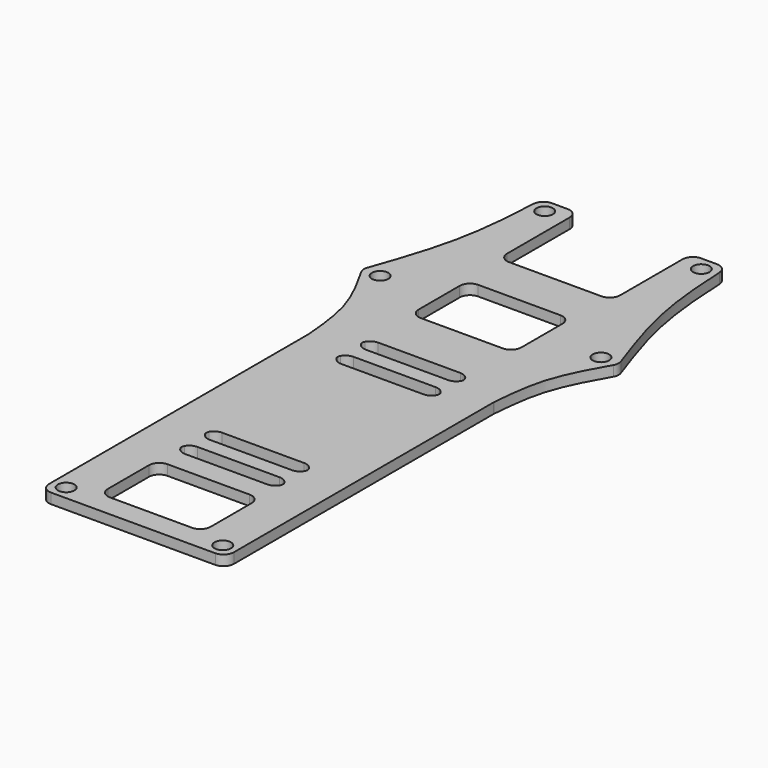
from build123d import *

# Parameters (mm, degrees)
F0_R          = 1.6
F0_W          = 20
F0_H          = 3
F0_H_2        = 14
F0_W_2        = 36
F0_H_3        = 50
F1_DEPTH      = 2
F2_T3_DEPTH   = 12
F2_T6_DEPTH   = 12
F2_T9_DEPTH   = 11.4916492708
F2_T12_DEPTH  = 11.4916492708
F2_T15_DEPTH  = 12
F2_T18_DEPTH  = 12
F2_T21_DEPTH  = 6.5584053931
F2_T24_DEPTH  = 6.5584053931
F2_T28_DEPTH  = 2
F2_T31_DEPTH  = 2
F2_T34_DEPTH  = 2
F2_T37_DEPTH  = 2
F2_T40_DEPTH  = 2
F2_T43_DEPTH  = 2
F2_T46_DEPTH  = 2
F2_T49_DEPTH  = 2
F2_T52_DEPTH  = 2
F2_T55_DEPTH  = 2
F2_T58_DEPTH  = 2
F2_T61_DEPTH  = 2
F2_T64_DEPTH  = 2
F2_T67_DEPTH  = 2
F2_T70_DEPTH  = 2
F2_T73_DEPTH  = 2
F2_T76_DEPTH  = 2
F2_T79_DEPTH  = 2
F2_T82_DEPTH  = 2
F2_T85_DEPTH  = 2
F2_T88_DEPTH  = 2
F2_T91_DEPTH  = 2
F2_T94_DEPTH  = 2
F2_T97_DEPTH  = 2
F2_T100_DEPTH = 2
F2_T103_DEPTH = 2
F2_T106_DEPTH = 2
F2_T109_DEPTH = 2
F3_R          = 1


# Not quite as in the source:
# - a fillet or chamfer that OpenCascade refuses, or shapes differently, is made with other operations: its cross-section is extruded or revolved along the edge and cut away or added
# - a feature names something its author has since deleted; it is built from what else it names


with BuildPart() as f1:
    # F0 (on Top) → F1 (new body)
    with BuildSketch(Plane.XY):
        Polygon((-11, 72), (-18, 72), (-18, 15.25), (-18, 0), (18, 0), (18, 15.25), (18, 72), (11, 72), (11, 52.774557963), (-11, 52.774557963), align=None)
        with Locations((-15.25, 69.25)):
            Circle(F0_R, mode=Mode.SUBTRACT)
        with Locations((0, 12.15)):
            Rectangle(F0_W, F0_H, mode=Mode.SUBTRACT)
        with Locations((0, 18.15)):
            Rectangle(F0_W, F0_H, mode=Mode.SUBTRACT)
        with Locations((0, 37)):
            Rectangle(F0_W, F0_H_2, mode=Mode.SUBTRACT)
        with Locations((15.25, 69.25)):
            Circle(F0_R, mode=Mode.SUBTRACT)
        with BuildLine():
            Line((-18, 15.25), (-18, 72))
            add(Edge.make_bspline(
                [(-18, 72), (-18.3026254462, 66.1394008634), (-18.9136987258, 54.305447113), (-22.9583868009, 42.805008272), (-25, 37)],
                knots=[0, 0, 0, 0, 0.4952359338, 1, 1, 1, 1], degree=3))
            add(Edge.make_bspline(
                [(-25, 37), (-22.9586488257, 33.418624871), (-18.967687527, 26.4168263973), (-18.3175811324, 18.9147918612), (-18, 15.25)],
                knots=[0, 0, 0, 0, 0.511493603, 1, 1, 1, 1], degree=3))
        make_face()
        with Locations((-21.5, 37)):
            Circle(F0_R, mode=Mode.SUBTRACT)
        with Locations((0, -25)):
            Rectangle(F0_W_2, F0_H_3)
        with Locations((-15.25, -47.25)):
            Circle(F0_R, mode=Mode.SUBTRACT)
        Polygon((10, -45.65), (0, -45.65), (-10, -45.65), (-10, -31.65), (0, -31.65), (10, -31.65), align=None, mode=Mode.SUBTRACT)
        with Locations((0, -25.85)):
            Rectangle(F0_W, F0_H, mode=Mode.SUBTRACT)
        with Locations((0, -19.85)):
            Rectangle(F0_W, F0_H, mode=Mode.SUBTRACT)
        with Locations((15.25, -47.25)):
            Circle(F0_R, mode=Mode.SUBTRACT)
        with BuildLine():
            Line((18, 72), (18, 15.25))
            add(Edge.make_bspline(
                [(25, 37), (22.9586488257, 33.418624871), (18.967687527, 26.4168263973), (18.3175811324, 18.9147918612), (18, 15.25)],
                knots=[0, 0, 0, 0, 0.511493603, 1, 1, 1, 1], degree=3))
            add(Edge.make_bspline(
                [(18, 72), (18.3026254462, 66.1394008634), (18.9136987258, 54.305447113), (22.9583868009, 42.805008272), (25, 37)],
                knots=[0, 0, 0, 0, 0.4952359338, 1, 1, 1, 1], degree=3))
        make_face()
        with Locations((21.5, 37)):
            Circle(F0_R, mode=Mode.SUBTRACT)
    extrude(amount=F1_DEPTH)

    # F2: fillet of radius 2 on 36 edges, made by hand


with BuildPart() as f2_tool1:
    # F2_s2 → F2_t3 (new body)
    with BuildSketch(Plane.XY.offset(-5)):
        with BuildLine():
            ThreePointArc((13, 72), (11.5857864376, 71.4142135624), (11, 70))
            Line((11, 70), (11, 72))
            Line((11, 72), (13, 72))
        make_face()
    extrude(amount=F2_T3_DEPTH)


with BuildPart() as f2_tool4:
    # F2_s5 → F2_t6 (new body)
    with BuildSketch(Plane.XY.offset(-5)):
        with BuildLine():
            ThreePointArc((-13, 72), (-11.5857864376, 71.4142135624), (-11, 70))
            Line((-11, 70), (-11, 72))
            Line((-11, 72), (-13, 72))
        make_face()
    extrude(amount=F2_T6_DEPTH)


with BuildPart() as f2_tool7:
    # F2_s8 → F2_t9 (new body)
    with BuildSketch(Plane.XY.offset(-4.7458246354)):
        with BuildLine():
            ThreePointArc((-16.1016701458, 72), (-17.4777245293, 71.4513698129), (-18.0988339389, 70.1064743339))
            ThreePointArc((-18.0988339389, 70.1064743339), (-18.0490214969, 71.0532165802), (-18, 72))
            Line((-18, 72), (-16.1016701458, 72))
        make_face()
    extrude(amount=F2_T9_DEPTH)


with BuildPart() as f2_tool10:
    # F2_s11 → F2_t12 (new body)
    with BuildSketch(Plane.XY.offset(-4.7458246354)):
        with BuildLine():
            ThreePointArc((18.0988339389, 70.1064743339), (17.4777245293, 71.4513698129), (16.1016701458, 72))
            Line((16.1016701458, 72), (18, 72))
            ThreePointArc((18, 72), (18.0490214969, 71.0532165802), (18.0988339389, 70.1064743339))
        make_face()
    extrude(amount=F2_T12_DEPTH)


with BuildPart() as f2_tool13:
    # F2_s14 → F2_t15 (new body)
    with BuildSketch(Plane.XY.offset(-5)):
        with BuildLine():
            ThreePointArc((-18, -48), (-17.4142135624, -49.4142135624), (-16, -50))
            Line((-16, -50), (-18, -50))
            Line((-18, -50), (-18, -48))
        make_face()
    extrude(amount=F2_T15_DEPTH)


with BuildPart() as f2_tool16:
    # F2_s17 → F2_t18 (new body)
    with BuildSketch(Plane.XY.offset(-5)):
        with BuildLine():
            ThreePointArc((16, -50), (17.4142135624, -49.4142135624), (18, -48))
            Line((18, -48), (18, -50))
            Line((18, -50), (16, -50))
        make_face()
    extrude(amount=F2_T18_DEPTH)


with BuildPart() as f2_tool19:
    # F2_s20 → F2_t21 (new body)
    with BuildSketch(Plane.XY.offset(-2.2792026965)):
        with BuildLine():
            ThreePointArc((-24.697621668, 37.8600754231), (-24.8026656547, 37.0182702368), (-24.5493168148, 36.2086502171))
            ThreePointArc((-24.5493168148, 36.2086502171), (-24.774551113, 36.6043862268), (-25, 37))
            ThreePointArc((-25, 37), (-24.8487744639, 37.4300249237), (-24.697621668, 37.8600754231))
        make_face()
    extrude(amount=F2_T21_DEPTH)


with BuildPart() as f2_tool22:
    # F2_s23 → F2_t24 (new body)
    with BuildSketch(Plane.XY.offset(-2.2792026965)):
        with BuildLine():
            ThreePointArc((24.5493168148, 36.2086502171), (24.8026656547, 37.0182702368), (24.697621668, 37.8600754231))
            ThreePointArc((24.697621668, 37.8600754231), (24.8487744639, 37.4300249237), (25, 37))
            ThreePointArc((25, 37), (24.774551113, 36.6043862268), (24.5493168148, 36.2086502171))
        make_face()
    extrude(amount=F2_T24_DEPTH)


with BuildPart() as f1_1:
    add(f1.part)

    # F2_t25: cut F2_tool1, F2_tool4, F2_tool7, F2_tool10, F2_tool13, F2_tool16, F2_tool19, F2_tool22
    add([f2_tool1.part, f2_tool4.part, f2_tool7.part, f2_tool10.part, f2_tool13.part, f2_tool16.part, f2_tool19.part, f2_tool22.part], mode=Mode.SUBTRACT)


with BuildPart() as f2_tool26:
    # F2_s27 → F2_t28 (new body)
    with BuildSketch(Plane.XY):
        with BuildLine():
            ThreePointArc((-11, 54.774557963), (-10.4142135624, 53.3603444006), (-9, 52.774557963))
            Line((-9, 52.774557963), (-11, 52.774557963))
            Line((-11, 52.774557963), (-11, 54.774557963))
        make_face()
    extrude(amount=F2_T28_DEPTH)


with BuildPart() as f2_tool29:
    # F2_s30 → F2_t31 (new body)
    with BuildSketch(Plane.XY):
        with BuildLine():
            ThreePointArc((9, 52.774557963), (10.4142135624, 53.3603444006), (11, 54.774557963))
            Line((11, 54.774557963), (11, 52.774557963))
            Line((11, 52.774557963), (9, 52.774557963))
        make_face()
    extrude(amount=F2_T31_DEPTH)


with BuildPart() as f2_tool32:
    # F2_s33 → F2_t34 (new body)
    with BuildSketch(Plane.XY):
        with BuildLine():
            ThreePointArc((18.0074697855, 15.3361946129), (18.001868319, 15.2499281672), (18, 15.1635002466))
            Line((18, 15.1635002466), (18, 15.25))
            ThreePointArc((18, 15.25), (18.0037347479, 15.293097319), (18.0074697855, 15.3361946129))
        make_face()
    extrude(amount=F2_T34_DEPTH)


with BuildPart() as f2_tool35:
    # F2_s36 → F2_t37 (new body)
    with BuildSketch(Plane.XY):
        with BuildLine():
            ThreePointArc((-18, 15.1635002466), (-18.001868319, 15.2499281672), (-18.0074697855, 15.3361946129))
            ThreePointArc((-18.0074697855, 15.3361946129), (-18.0037347479, 15.293097319), (-18, 15.25))
            Line((-18, 15.25), (-18, 15.1635002466))
        make_face()
    extrude(amount=F2_T37_DEPTH)


with BuildPart() as f2_tool38:
    # F2_s39 → F2_t40 (new body)
    with BuildSketch(Plane.XY):
        with BuildLine():
            ThreePointArc((10, 11.65), (9.4142135624, 13.0642135624), (8, 13.65))
            Line((8, 13.65), (10, 13.65))
            Line((10, 13.65), (10, 11.65))
        make_face()
    extrude(amount=F2_T40_DEPTH)


with BuildPart() as f2_tool41:
    # F2_s42 → F2_t43 (new body)
    with BuildSketch(Plane.XY):
        with BuildLine():
            ThreePointArc((-8, 13.65), (-9.4142135624, 13.0642135624), (-10, 11.65))
            Line((-10, 11.65), (-10, 13.65))
            Line((-10, 13.65), (-8, 13.65))
        make_face()
    extrude(amount=F2_T43_DEPTH)


with BuildPart() as f2_tool44:
    # F2_s45 → F2_t46 (new body)
    with BuildSketch(Plane.XY):
        with BuildLine():
            ThreePointArc((-8, 10.65), (-9.4142135624, 11.2357864376), (-10, 12.65))
            Line((-10, 12.65), (-10, 10.65))
            Line((-10, 10.65), (-8, 10.65))
        make_face()
    extrude(amount=F2_T46_DEPTH)


with BuildPart() as f2_tool47:
    # F2_s48 → F2_t49 (new body)
    with BuildSketch(Plane.XY):
        with BuildLine():
            ThreePointArc((10, 12.65), (9.4142135624, 11.2357864376), (8, 10.65))
            Line((8, 10.65), (10, 10.65))
            Line((10, 10.65), (10, 12.65))
        make_face()
    extrude(amount=F2_T49_DEPTH)


with BuildPart() as f2_tool50:
    # F2_s51 → F2_t52 (new body)
    with BuildSketch(Plane.XY):
        with BuildLine():
            ThreePointArc((8, -24.35), (9.4142135624, -24.9357864376), (10, -26.35))
            Line((10, -26.35), (10, -24.35))
            Line((10, -24.35), (8, -24.35))
        make_face()
    extrude(amount=F2_T52_DEPTH)


with BuildPart() as f2_tool53:
    # F2_s54 → F2_t55 (new body)
    with BuildSketch(Plane.XY):
        with BuildLine():
            ThreePointArc((-8, -24.35), (-9.4142135624, -24.9357864376), (-10, -26.35))
            Line((-10, -26.35), (-10, -24.35))
            Line((-10, -24.35), (-8, -24.35))
        make_face()
    extrude(amount=F2_T55_DEPTH)


with BuildPart() as f2_tool56:
    # F2_s57 → F2_t58 (new body)
    with BuildSketch(Plane.XY):
        with BuildLine():
            ThreePointArc((-10, -25.35), (-9.4142135624, -26.7642135624), (-8, -27.35))
            Line((-8, -27.35), (-10, -27.35))
            Line((-10, -27.35), (-10, -25.35))
        make_face()
    extrude(amount=F2_T58_DEPTH)


with BuildPart() as f2_tool59:
    # F2_s60 → F2_t61 (new body)
    with BuildSketch(Plane.XY):
        with BuildLine():
            ThreePointArc((10, -25.35), (9.4142135624, -26.7642135624), (8, -27.35))
            Line((8, -27.35), (10, -27.35))
            Line((10, -27.35), (10, -25.35))
        make_face()
    extrude(amount=F2_T61_DEPTH)


with BuildPart() as f2_tool62:
    # F2_s63 → F2_t64 (new body)
    with BuildSketch(Plane.XY):
        with BuildLine():
            ThreePointArc((-10, -33.65), (-9.4142135624, -32.2357864376), (-8, -31.65))
            Line((-8, -31.65), (-10, -31.65))
            Line((-10, -31.65), (-10, -33.65))
        make_face()
    extrude(amount=F2_T64_DEPTH)


with BuildPart() as f2_tool65:
    # F2_s66 → F2_t67 (new body)
    with BuildSketch(Plane.XY):
        with BuildLine():
            ThreePointArc((10, -33.65), (9.4142135624, -32.2357864376), (8, -31.65))
            Line((8, -31.65), (10, -31.65))
            Line((10, -31.65), (10, -33.65))
        make_face()
    extrude(amount=F2_T67_DEPTH)


with BuildPart() as f2_tool68:
    # F2_s69 → F2_t70 (new body)
    with BuildSketch(Plane.XY):
        with BuildLine():
            ThreePointArc((8, -45.65), (9.4142135624, -45.0642135624), (10, -43.65))
            Line((10, -43.65), (10, -45.65))
            Line((10, -45.65), (8, -45.65))
        make_face()
    extrude(amount=F2_T70_DEPTH)


with BuildPart() as f2_tool71:
    # F2_s72 → F2_t73 (new body)
    with BuildSketch(Plane.XY):
        with BuildLine():
            ThreePointArc((-8, -45.65), (-9.4142135624, -45.0642135624), (-10, -43.65))
            Line((-10, -43.65), (-10, -45.65))
            Line((-10, -45.65), (-8, -45.65))
        make_face()
    extrude(amount=F2_T73_DEPTH)


with BuildPart() as f2_tool74:
    # F2_s75 → F2_t76 (new body)
    with BuildSketch(Plane.XY):
        with BuildLine():
            ThreePointArc((-8, 19.65), (-9.4142135624, 19.0642135624), (-10, 17.65))
            Line((-10, 17.65), (-10, 19.65))
            Line((-10, 19.65), (-8, 19.65))
        make_face()
    extrude(amount=F2_T76_DEPTH)


with BuildPart() as f2_tool77:
    # F2_s78 → F2_t79 (new body)
    with BuildSketch(Plane.XY):
        with BuildLine():
            ThreePointArc((-10, 18.65), (-9.4142135624, 17.2357864376), (-8, 16.65))
            Line((-8, 16.65), (-10, 16.65))
            Line((-10, 16.65), (-10, 18.65))
        make_face()
    extrude(amount=F2_T79_DEPTH)


with BuildPart() as f2_tool80:
    # F2_s81 → F2_t82 (new body)
    with BuildSketch(Plane.XY):
        with BuildLine():
            ThreePointArc((-8, -21.35), (-9.4142135624, -20.7642135624), (-10, -19.35))
            Line((-10, -19.35), (-10, -21.35))
            Line((-10, -21.35), (-8, -21.35))
        make_face()
    extrude(amount=F2_T82_DEPTH)


with BuildPart() as f2_tool83:
    # F2_s84 → F2_t85 (new body)
    with BuildSketch(Plane.XY):
        with BuildLine():
            ThreePointArc((-8, -18.35), (-9.4142135624, -18.9357864376), (-10, -20.35))
            Line((-10, -20.35), (-10, -18.35))
            Line((-10, -18.35), (-8, -18.35))
        make_face()
    extrude(amount=F2_T85_DEPTH)


with BuildPart() as f2_tool86:
    # F2_s87 → F2_t88 (new body)
    with BuildSketch(Plane.XY):
        with BuildLine():
            ThreePointArc((10, -20.35), (9.4142135624, -18.9357864376), (8, -18.35))
            Line((8, -18.35), (10, -18.35))
            Line((10, -18.35), (10, -20.35))
        make_face()
    extrude(amount=F2_T88_DEPTH)


with BuildPart() as f2_tool89:
    # F2_s90 → F2_t91 (new body)
    with BuildSketch(Plane.XY):
        with BuildLine():
            ThreePointArc((10, -19.35), (9.4142135624, -20.7642135624), (8, -21.35))
            Line((8, -21.35), (10, -21.35))
            Line((10, -21.35), (10, -19.35))
        make_face()
    extrude(amount=F2_T91_DEPTH)


with BuildPart() as f2_tool92:
    # F2_s93 → F2_t94 (new body)
    with BuildSketch(Plane.XY):
        with BuildLine():
            ThreePointArc((10, 18.65), (9.4142135624, 17.2357864376), (8, 16.65))
            Line((8, 16.65), (10, 16.65))
            Line((10, 16.65), (10, 18.65))
        make_face()
    extrude(amount=F2_T94_DEPTH)


with BuildPart() as f2_tool95:
    # F2_s96 → F2_t97 (new body)
    with BuildSketch(Plane.XY):
        with BuildLine():
            ThreePointArc((8, 19.65), (9.4142135624, 19.0642135624), (10, 17.65))
            Line((10, 17.65), (10, 19.65))
            Line((10, 19.65), (8, 19.65))
        make_face()
    extrude(amount=F2_T97_DEPTH)


with BuildPart() as f2_tool98:
    # F2_s99 → F2_t100 (new body)
    with BuildSketch(Plane.XY):
        with BuildLine():
            ThreePointArc((-8, 44), (-9.4142135624, 43.4142135624), (-10, 42))
            Line((-10, 42), (-10, 44))
            Line((-10, 44), (-8, 44))
        make_face()
    extrude(amount=F2_T100_DEPTH)


with BuildPart() as f2_tool101:
    # F2_s102 → F2_t103 (new body)
    with BuildSketch(Plane.XY):
        with BuildLine():
            ThreePointArc((8, 44), (9.4142135624, 43.4142135624), (10, 42))
            Line((10, 42), (10, 44))
            Line((10, 44), (8, 44))
        make_face()
    extrude(amount=F2_T103_DEPTH)


with BuildPart() as f2_tool104:
    # F2_s105 → F2_t106 (new body)
    with BuildSketch(Plane.XY):
        with BuildLine():
            ThreePointArc((10, 32), (9.4142135624, 30.5857864376), (8, 30))
            Line((8, 30), (10, 30))
            Line((10, 30), (10, 32))
        make_face()
    extrude(amount=F2_T106_DEPTH)


with BuildPart() as f2_tool107:
    # F2_s108 → F2_t109 (new body)
    with BuildSketch(Plane.XY):
        with BuildLine():
            ThreePointArc((-10, 32), (-9.4142135624, 30.5857864376), (-8, 30))
            Line((-8, 30), (-10, 30))
            Line((-10, 30), (-10, 32))
        make_face()
    extrude(amount=F2_T109_DEPTH)


with BuildPart() as f1_2:
    add(f1_1.part)

    # F2_t110: union F2_tool26, F2_tool29, F2_tool32, F2_tool35, F2_tool38, F2_tool41, F2_tool44, F2_tool47, F2_tool50, F2_tool53, F2_tool56, F2_tool59, F2_tool62, F2_tool65, F2_tool68, F2_tool71, F2_tool74, F2_tool77, F2_tool80, F2_tool83, F2_tool86, F2_tool89, F2_tool92, F2_tool95, F2_tool98, F2_tool101, F2_tool104, F2_tool107
    add([f2_tool26.part, f2_tool29.part, f2_tool32.part, f2_tool35.part, f2_tool38.part, f2_tool41.part, f2_tool44.part, f2_tool47.part, f2_tool50.part, f2_tool53.part, f2_tool56.part, f2_tool59.part, f2_tool62.part, f2_tool65.part, f2_tool68.part, f2_tool71.part, f2_tool74.part, f2_tool77.part, f2_tool80.part, f2_tool83.part, f2_tool86.part, f2_tool89.part, f2_tool92.part, f2_tool95.part, f2_tool98.part, f2_tool101.part, f2_tool104.part, f2_tool107.part])

    # F3
    f3_edges = [f1_2.edges().sort_by_distance(p)[0] for p in [
        (-9.936492, -25.85, 1),
        (9.936492, -25.85, 1),
        (9.936492, 12.15, 1),
        (-9.936492, 12.15, 1),
        (9.936492, 18.15, 1),
        (-9.936492, 18.15, 1),
        (-9.936492, -19.85, 1),
        (9.936492, -19.85, 1),
    ]]
    fillet(f3_edges, radius=F3_R)


solid = f1_2.part
